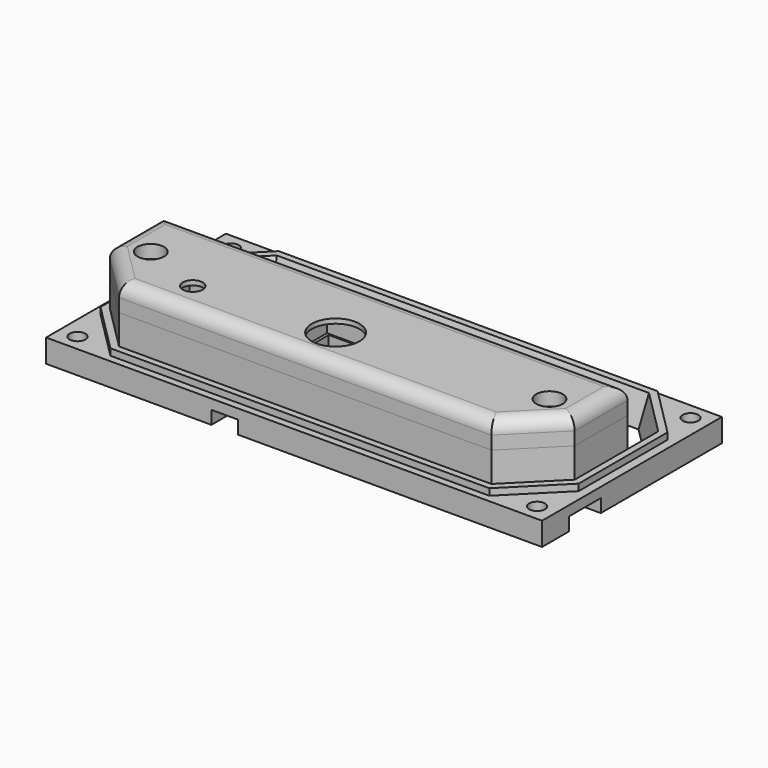
from build123d import *

# Parameters (mm, degrees)
F0_W            = 75
F0_H            = 34
F0_R            = 1.2
F1_DEPTH        = 3.5
F3_DEPTH        = 1
F5_DEPTH        = 5
F11_DEPTH       = 9
F12_W           = 15
F12_H           = 10
F13_DEPTH       = 8.5
F14_W           = 7.3
F14_H           = 4.5
F15_DEPTH       = 5
F16_W           = 9
F16_H           = 10
F16_W_2         = 7
F16_H_2         = 4
F17_DEPTH       = 25
F18_W           = 2
F18_H           = 5
F19_DEPTH       = 10
F20_W           = 6
F20_H           = 2
F21_DEPTH       = 25
F22_R           = 0.8
F23_DEPTH       = 5
F26_DEPTH       = 4
F27_R           = 3.6
F27_R_2         = 1.5
F28_DEPTH       = 25
F29_W           = 13
F29_H           = 10.5
F29_W_2         = 8
F29_H_2         = 5
F30_DEPTH       = 3.3
F31_W           = 2
F31_H           = 4
F32_DEPTH       = 7
F33_W           = 4
F33_H           = 2
F34_DEPTH       = 25
F36_D           = 2
F36_DEPTH       = 10
F36_CBORE_D     = 4
F36_CBORE_DEPTH = 2
F36_TIP         = 0.600860619
F37_R           = 2


with BuildPart() as f1:
    # F0 (on Top) → F1 (new body)
    with BuildSketch(Plane.XY):
        Rectangle(F0_W, F0_H)
        with Locations((-34.75, -14.5)):
            Circle(F0_R, mode=Mode.SUBTRACT)
        with Locations((34.75, -14.5)):
            Circle(F0_R, mode=Mode.SUBTRACT)
        with Locations((-34.75, 14.5)):
            Circle(F0_R, mode=Mode.SUBTRACT)
        with Locations((34.75, 14.5)):
            Circle(F0_R, mode=Mode.SUBTRACT)
    extrude(amount=F1_DEPTH)

    # F2 (on face) → F3 (join)
    with BuildSketch(Plane.XY.offset(3.5)):
        Polygon((28.65, 15.9), (-28.65, 15.9), (-36.15, 8.4), (-36.15, -8.4), (-28.65, -15.9), (28.65, -15.9), (36.15, -8.4), (36.15, 8.4), align=None)
    extrude(amount=F3_DEPTH)

    # F4 (on face) → F5 (cut)
    with BuildSketch(Plane.XY.offset(4.5)):
        Polygon((28.15, 14.9), (-28.15, 14.9), (-35.15, 7.9), (-35.15, -7.9), (-28.15, -14.9), (28.15, -14.9), (35.15, -7.9), (35.15, 7.9), align=None)
    extrude(amount=-F5_DEPTH, mode=Mode.SUBTRACT)

    # F9: sweep along a path in F8
    with BuildLine(Plane.XY.offset(4.5)) as f9_path:
        Line((-35.15, 2.1), (-35.15, 7.9))
        Line((-35.15, 7.9), (-28.15, 14.9))
        Line((-28.15, 14.9), (28.15, 14.9))
        Line((28.15, 14.9), (35.15, 7.9))
        Line((35.15, 7.9), (35.15, 2.1))
    # F7 (on offset) → F9 (sweep)
    with BuildSketch(Plane.XZ.offset(-2.1)):
        Polygon((-33.85, 0), (-35.15, 4.5), (-35.15, 0), align=None)
    sweep(path=f9_path.line, transition=Transition.RIGHT)

    # F10 (on Top) → F11 (join)
    with BuildSketch(Plane.XY):
        Polygon((-35.15, -7.9), (-28.15, -14.9), (28.15, -14.9), (35.15, -7.9), (35.15, 2.1), (-35.15, 2.1), align=None)
    extrude(amount=F11_DEPTH)

    # F12 (on face) → F13 (cut)
    with BuildSketch(Plane.XY.offset(9)):
        with Locations((2.25, -8.9)):
            Rectangle(F12_W, F12_H)
    extrude(amount=-F13_DEPTH, mode=Mode.SUBTRACT)

    # F14 (on face) → F15 (cut)
    with BuildSketch(Plane.XY.offset(9)):
        with Locations((-19.15, -10.15)):
            Rectangle(F14_W, F14_H)
    extrude(amount=-F15_DEPTH, mode=Mode.SUBTRACT)

    # F16 (on face) → F17 (cut)
    with BuildSketch(Plane.XY.offset(9)):
        with Locations((14.25, -8.9)):
            Rectangle(F16_W, F16_H)
        with Locations((-12, -10.15)):
            Rectangle(F16_W_2, F16_H_2)
    extrude(amount=-F17_DEPTH, mode=Mode.SUBTRACT)

    # F18 (on face) → F19 (join)
    with BuildSketch(Plane.XZ.offset(3.9)):
        with Locations((15.25, 2.5)):
            Rectangle(F18_W, F18_H)
    extrude(amount=F19_DEPTH)

    # F20 (on face) → F21 (cut)
    with BuildSketch(Plane(origin=(14.25, 0, 0), x_dir=(0, -1, 0), z_dir=(-1, 0, 0))):
        with Locations((8.9, 1)):
            Rectangle(F20_W, F20_H)
    extrude(amount=-F21_DEPTH, mode=Mode.SUBTRACT)

    # F22 (on face) → F23 (cut)
    with BuildSketch(Plane.XY.offset(9)):
        with Locations((-30.15, -6.4)):
            Circle(F22_R)
        with Locations((30.15, -6.4)):
            Circle(F22_R)
    extrude(amount=-F23_DEPTH, mode=Mode.SUBTRACT)

    # F31 (on face) → F32 (join)
    with BuildSketch(Plane.YZ.offset(-15.5)):
        with Locations((-10.15, 2)):
            Rectangle(F31_W, F31_H)
    extrude(amount=F32_DEPTH)

    # F33 (on face) → F34 (cut)
    with BuildSketch(Plane(origin=(0, -9.15, 0), x_dir=(-1, 0, 0), z_dir=(0, 1, 0))):
        with Locations((10.5, 1)):
            Rectangle(F33_W, F33_H)
    extrude(amount=-F34_DEPTH, mode=Mode.SUBTRACT)


with BuildPart() as f26:
    # F25 (on offset) → F26 (new body)
    with BuildSketch(Plane.XY.offset(9)):
        Polygon((-35.15, -7.9), (-28.15, -14.9), (28.15, -14.9), (35.15, -7.9), (35.15, 2.1), (-35.15, 2.1), align=None)
    extrude(amount=F26_DEPTH)

    # F27 (on face) → F28 (cut)
    with BuildSketch(Plane.XY.offset(13)):
        with Locations((-0.2, -8.9)):
            Circle(F27_R)
        with Locations((-20.8, -10.15)):
            Circle(F27_R_2)
    extrude(amount=-F28_DEPTH, mode=Mode.SUBTRACT)

    # F29 (on face) → F30 (cut)
    with BuildSketch(Plane(origin=(0, 0, 9), x_dir=(1, 0, 0), z_dir=(0, 0, -1))):
        with Locations((0.8, 8.9)):
            Rectangle(F29_W, F29_H)
        with Locations((-19.3, 10.15)):
            Rectangle(F29_W_2, F29_H_2)
    extrude(amount=-F30_DEPTH, mode=Mode.SUBTRACT)

    # F36
    with Locations(Plane.XY.offset(13)):
        with Locations((-30.15, -6.4), (30.15, -6.4)):
            CounterBoreHole(F36_D / 2, F36_CBORE_D / 2, F36_CBORE_DEPTH, depth=F36_DEPTH)
            with Locations((0, 0, -(F36_DEPTH + F36_TIP / 2))):  # 118° drill point
                Cone(0, F36_D / 2, F36_TIP, mode=Mode.SUBTRACT)

    # F37
    f37_edges = [f26.edges().sort_by_distance(p)[0] for p in [
        (0, -14.9, 13),
        (-31.65, -11.4, 13),
        (-35.15, -2.9, 13),
        (0, 2.1, 13),
        (35.15, -2.9, 13),
        (31.65, -11.4, 13),
    ]]
    fillet(f37_edges, radius=F37_R)


solid = Compound([f1.part, f26.part])
